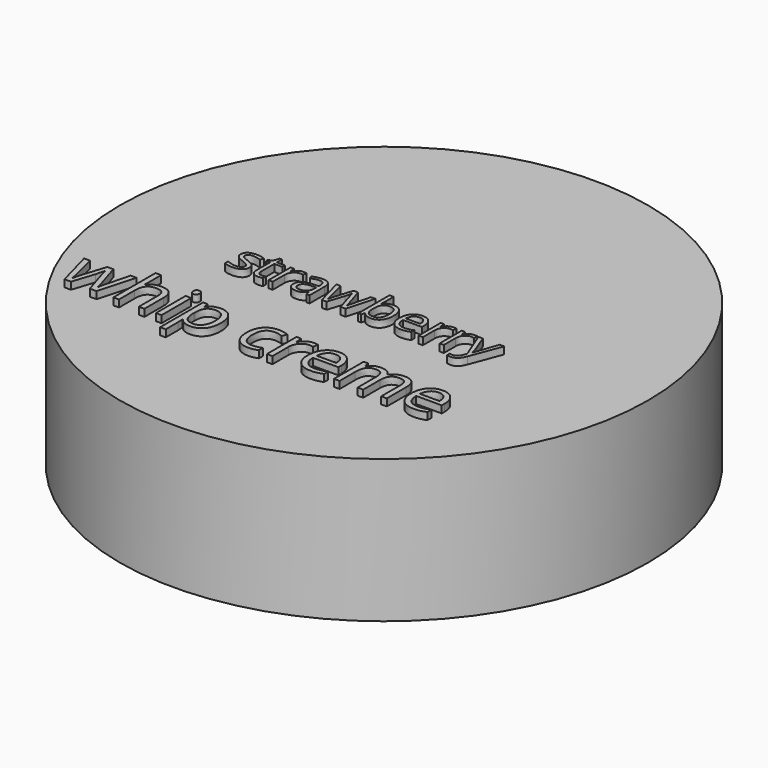
from build123d import *

# Parameters (mm, degrees)
F0_R         = 9.3932902921
F1_DEPTH     = 5.08
F3_TEXT_SIZE = 2.4630972702
F2_TEXT_SIZE = 1.8309775947
F4_DEPTH     = 0.254


# Not quite as in the source:
# - Text() gives the source's letters only with a copy of the font that has no kerning and outlines rounded to 1/6400 em; it was checked with that copy


with BuildPart() as f1:
    # F0 (on Top) → F1 (new body)
    with BuildSketch(Plane.XY):
        Circle(F0_R)
    extrude(amount=-F1_DEPTH)

    # F3 (on face) + F2 (on face) → F4 (join)
    with BuildSketch(Plane.XY):
        with Locations((-7.8978128731, -4.8156585544)):
            Text('whip creme', F3_TEXT_SIZE, font='Open Sans', text_align=(TextAlign.LEFT, TextAlign.BOTTOM))
    with BuildSketch(Plane.XY):
        with Locations((-4.7296388051, -1.3183038682)):
            Text('strawberry', F2_TEXT_SIZE, font='Open Sans', text_align=(TextAlign.LEFT, TextAlign.BOTTOM))
    extrude(amount=F4_DEPTH)


solid = f1.part
